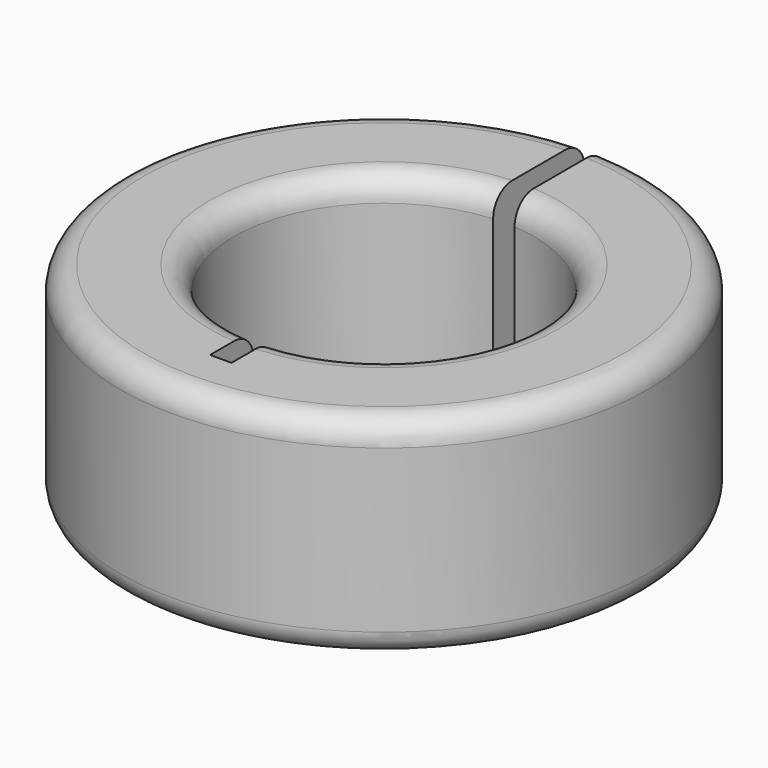
from build123d import *

# Parameters (mm, degrees)
F1_DEPTH = 11.1125
F2_R     = 1.27


# Not quite as in the source:
# - a feature names something its author has since deleted; it is built from what else it names


with BuildPart() as f1:
    # F0 (on Top) → F1 (new body)
    with BuildSketch(Plane.XY):
        with BuildLine():
            Line((0.5669642458, -7.9299578551), (0.5669642458, -10.7905164226))
            Line((0.5669642458, -10.7905164226), (-0.5669642458, -10.7905164226))
            Line((-0.5669642458, -10.7905164226), (-0.5669642458, -7.9299578551))
            ThreePointArc((-0.5669642458, -7.9299578551), (-7.950199987, -0.0004547511), (-0.5678714286, 7.9298929426))
            Line((-0.5678714286, 7.9298929426), (-0.5678714286, 13.9584534258))
            ThreePointArc((-0.5678714286, 13.9584534258), (0.0009078918, -13.9699999705), (0.566057141, 13.9585271183))
            Line((0.566057141, 13.9585271183), (0.566057141, 7.9300226578))
            ThreePointArc((0.566057141, 7.9300226578), (7.950199987, 0.0004547083), (0.5669642458, -7.9299578551))
        make_face()
    extrude(amount=F1_DEPTH)

    # F2
    f2_edges = [f1.edges().sort_by_distance(p)[0] for p in [
        (-7.9502, -0.000455, 11.1125),
        (-7.9502, -0.000455, 0),
        (0.000908, -13.97, 11.1125),
        (0.000908, -13.97, 0),
        (7.9502, 0.000455, 11.1125),
        (7.9502, 0.000455, 0),
    ]]
    fillet(f2_edges, radius=F2_R)


solid = f1.part
